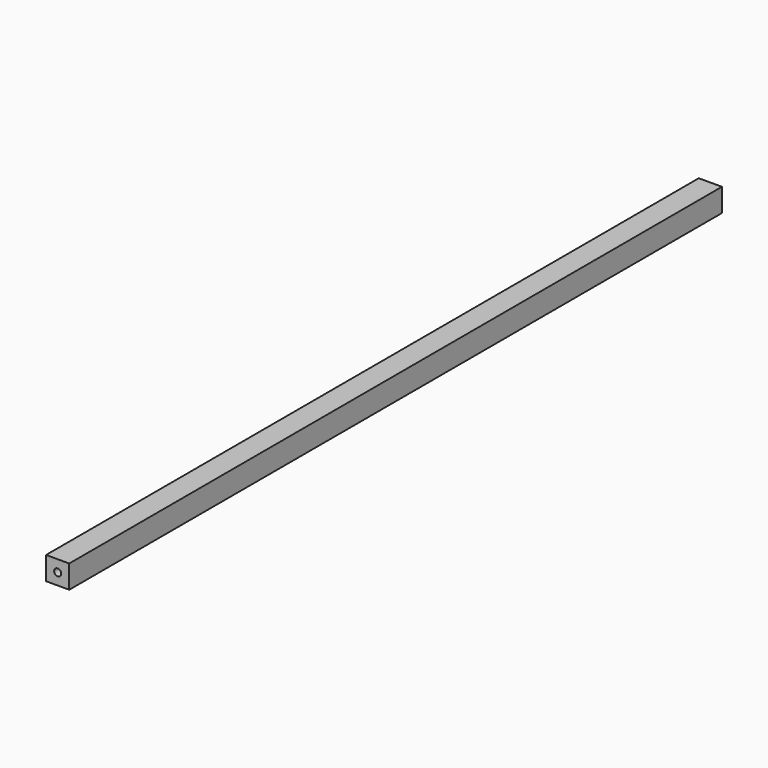
from build123d import *

# Parameters (mm, degrees)
F0_W     = 20
F0_H     = 20
F1_DEPTH = 352.4825
F2_R     = 3
F3_DEPTH = 12
F4_R     = 3
F5_DEPTH = 12


with BuildPart() as f1:
    # F0 (on Front) → F1 (new body, symmetric)
    with BuildSketch(Plane.XZ):
        with Locations((10, 10)):
            Rectangle(F0_W, F0_H)
    extrude(amount=F1_DEPTH, both=True)

    # F2 (on face) → F3 (cut)
    with BuildSketch(Plane.XZ.offset(352.4825)):
        with Locations((10, 10)):
            Circle(F2_R)
    extrude(amount=-F3_DEPTH, mode=Mode.SUBTRACT)

    # F4 (on face) → F5 (cut)
    with BuildSketch(Plane(origin=(0, 352.4825, 0), x_dir=(-1, 0, 0), z_dir=(0, 1, 0))):
        with Locations((-10, 10)):
            Circle(F4_R)
    extrude(amount=-F5_DEPTH, mode=Mode.SUBTRACT)


solid = f1.part
